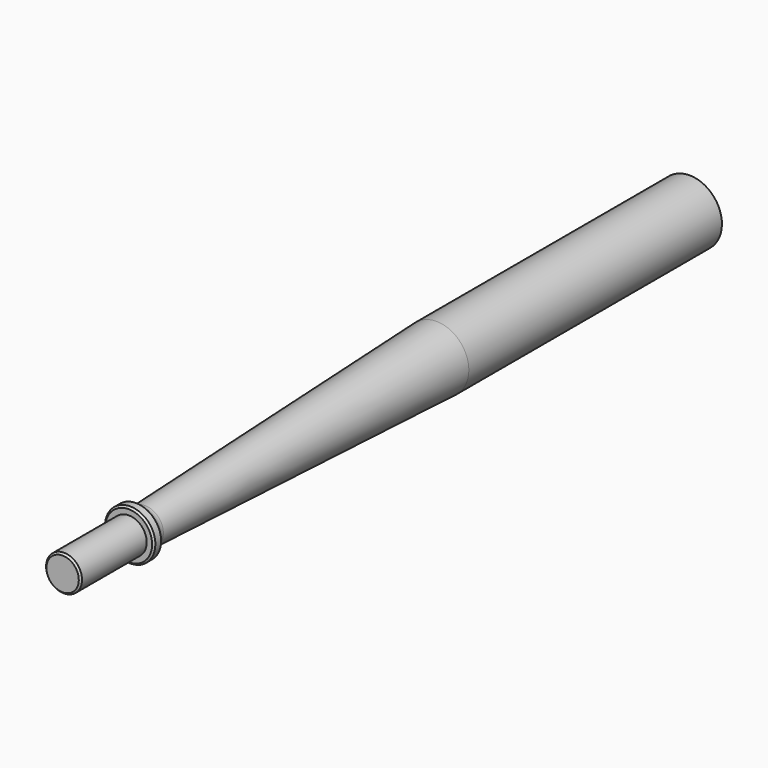
from build123d import *

# Parameters (mm, degrees)
F2_R     = 6
F3_DEPTH = 100
F4_SIZE  = 0.5


# Not quite as in the source:
# - a fillet or chamfer that OpenCascade refuses, or shapes differently, is made with other operations: its cross-section is extruded or revolved along the edge and cut away or added


with BuildPart() as f1:
    # F0 (on Right) → F1 (revolve)
    with BuildSketch(Plane.YZ):
        Polygon((108.9967988729, 0), (108.9967988729, 9), (20.9967988729, 9), (-83.0032011271, 5), (-83.0032011271, 7), (-86.0032011271, 7), (-86.0032011271, 5), (-109.0032011271, 5), (-109.0032011271, 0), align=None)
    revolve(axis=Axis((0, -0.0032011271, 0), (0, -1, 0)))

    # F2 (on face) → F3 (cut)
    with BuildSketch(Plane(origin=(0, 108.9967988729, 0), x_dir=(-1, 0, 0), z_dir=(0, 1, 0))):
        Circle(F2_R)
    extrude(amount=-F3_DEPTH, mode=Mode.SUBTRACT)

    # F4
    f4_edges = [f1.edges().sort_by_distance(p)[0] for p in [
        (0, -109.003201, -5),
        (0, -83.003201, -7),
        (0, -86.003201, -7),
    ]]
    chamfer(f4_edges, length=F4_SIZE)

    # F5: fillet of radius 3 on 1 edges, made by hand

    # F5_s1 → F5_t2 (revolve)
    with BuildSketch(Plane.YZ):
        with BuildLine():
            ThreePointArc((-83.0032011271, 6.5), (-81.8638498753, 5.4457220241), (-80.350077034, 5.1020432343))
            Line((-80.350077034, 5.1020432343), (-80.3477710467, 5.0420875639))
            Line((-80.3477710467, 5.0420875639), (-83.0008951397, 4.9400443295))
            Line((-83.0008951397, 4.9400443295), (-83.0632011271, 5))
            ThreePointArc((-83.0632011271, 5), (-83.0632011271, 5.75), (-83.0539576216, 6.4680034648))
            Line((-83.0539576216, 6.4680034648), (-83.0032011271, 6.5))
        make_face()
    revolve(axis=Axis((0, -83.0032011271, 0), (0, -1, 0)))


solid = f1.part
